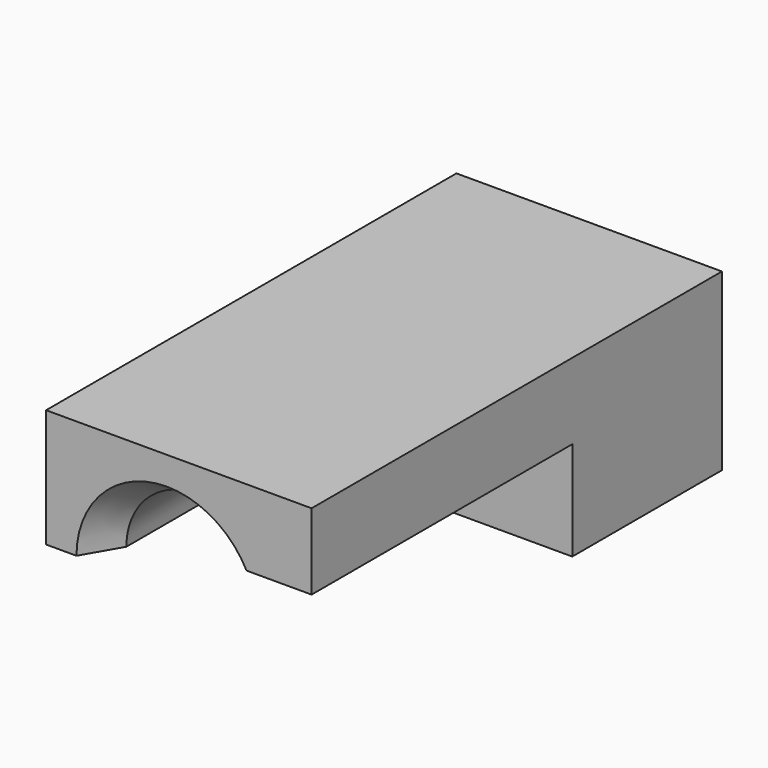
from build123d import *

# Parameters (mm, degrees)
F0_R     = 1.62
F0_R_2   = 2
F1_DEPTH = 15.5
F3_DEPTH = 27
F4_D     = 4
F4_DEPTH = 8
F4_TIP   = 1.2017212381
F5_DEPTH = 6
F6_SIZE2 = 1.7320508076
F6_SIZE  = 3


# Not quite as in the source:
# - ends of sketch curves that miss each other by under 0.0002 mm in the source are joined


with BuildPart() as f1:
    # F0 (on Front) → F1 (new body)
    with BuildSketch(Plane.XZ):
        with BuildLine():
            Line((-81.938941, 0.95), (-79.867763328, 0.95))
            ThreePointArc((-79.867763328, 0.95), (-84.599863166, 4.7050416476), (-90.5653650686, 3.7532564808))
            ThreePointArc((-90.5653650686, 3.7532564808), (-90.517166249, 3.503677095), (-90.501013, 3.25))
            ThreePointArc((-90.501013, 3.25), (-91.2509614327, 1.6887917887), (-92.9383840791, 1.2984092286))
            ThreePointArc((-92.9383840791, 1.2984092286), (-93.5417590804, 0.0341622689), (-93.899505073, -1.3202378094))
            ThreePointArc((-93.899505073, -1.3202378094), (-93.0082544766, -0.8153925244), (-91.9839548989, -0.8179930331))
            ThreePointArc((-91.9839548989, -0.8179930331), (-87.4977327048, 3.112954161), (-81.938941, 0.95))
        make_face()
        with BuildLine():
            ThreePointArc((-90.5653650686, 3.7532564808), (-84.599863166, 4.7050416476), (-79.867763328, 0.9499998269))
            Line((-79.867763328, 0.9499998269), (-74.501013, 0.95))
            Line((-74.501013, 0.95), (-74.501013, 7.25))
            Line((-74.501013, 7.25), (-96.501013, 7.25))
            Line((-96.501013, 7.25), (-96.501013, -2.55))
            Line((-96.501013, -2.55), (-94.4909878742, -2.55))
            ThreePointArc((-94.4909878742, -2.55), (-94.3033741804, -1.8831123628), (-93.899505073, -1.3202378094))
            ThreePointArc((-93.899505073, -1.3202378094), (-93.5417590804, 0.0341622689), (-92.9383840791, 1.2984092286))
            ThreePointArc((-92.9383840791, 1.2984092286), (-93.9389897521, 4.6400441937), (-90.5653650686, 3.7532564808))
        make_face()
        with Locations((-78.501013, 3.25)):
            Circle(F0_R, mode=Mode.SUBTRACT)
        with BuildLine():
            Line((-74.501013, 0.95), (-79.867763328, 0.95))
            Line((-79.867763328, 0.95), (-81.938941, 0.95))
            ThreePointArc((-81.9389410644, 0.9499999506), (-87.4977327048, 3.112954161), (-91.9839548989, -0.8179930331))
            ThreePointArc((-91.9839548989, -0.8179930331), (-92.0381964068, -1.0001290636), (-92.086389397, -1.1839580887))
            ThreePointArc((-92.086389397, -1.1839580887), (-91.2172509043, -1.7618932843), (-90.881013, -2.75))
            ThreePointArc((-90.881013, -2.75), (-92.6012048017, -4.3668987609), (-94.1086199171, -2.55))
            Line((-94.1086199171, -2.55), (-94.4909878742, -2.55))
            Line((-94.4909878742, -2.55), (-96.501013, -2.55))
            Line((-96.501013, -2.55), (-96.501013, -7.25))
            Line((-96.501013, -7.25), (-74.501013, -7.25))
            Line((-74.501013, -7.25), (-74.501013, 0.95))
        make_face()
        with Locations((-78.501013, -2.75)):
            Circle(F0_R_2, mode=Mode.SUBTRACT)
        with BuildLine():
            ThreePointArc((-92.9383840791, 1.2984092286), (-91.8934258204, 2.6626657264), (-90.5653650686, 3.7532564808))
            ThreePointArc((-90.5653650686, 3.7532564808), (-93.9389897521, 4.6400441937), (-92.9383840791, 1.2984092286))
        make_face()
        with Locations((-78.501013, -2.75)):
            Circle(F0_R_2)
        with BuildLine():
            ThreePointArc((-90.501013, 3.25), (-90.517166249, 3.503677095), (-90.5653650686, 3.7532564808))
            ThreePointArc((-90.5653650686, 3.7532564808), (-91.8934258204, 2.6626657264), (-92.9383840791, 1.2984092286))
            ThreePointArc((-92.9383840791, 1.2984092286), (-91.2509614327, 1.6887917887), (-90.501013, 3.25))
        make_face()
        with Locations((-78.501013, 3.25)):
            Circle(F0_R)
        with BuildLine():
            ThreePointArc((-93.9879149105, -2.1069426863), (-93.9540972375, -1.7124229299), (-93.899505073, -1.3202378094))
            ThreePointArc((-93.899505073, -1.3202378094), (-94.3033741804, -1.8831123628), (-94.4909878742, -2.55))
            Line((-94.4909878742, -2.55), (-94.1086199171, -2.55))
            ThreePointArc((-94.1086199171, -2.55), (-94.0640456826, -2.324172766), (-93.9879149105, -2.1069426863))
        make_face()
        with BuildLine():
            ThreePointArc((-92.086389397, -1.1839580887), (-92.0381964068, -1.0001290636), (-91.9839548989, -0.8179930331))
            ThreePointArc((-91.9839548989, -0.8179930331), (-93.0082544766, -0.8153925244), (-93.899505073, -1.3202378094))
            ThreePointArc((-93.899505073, -1.3202378094), (-93.9540972375, -1.7124229299), (-93.9879149105, -2.1069426863))
            ThreePointArc((-93.9879149105, -2.1069426863), (-93.2084169398, -1.29261204), (-92.086389397, -1.1839580887))
        make_face()
        with BuildLine():
            ThreePointArc((-90.881013, -2.75), (-91.2172509043, -1.7618932843), (-92.086389397, -1.1839580887))
            ThreePointArc((-92.086389397, -1.1839580887), (-92.2097087478, -1.8620371678), (-92.251013, -2.55))
            Line((-92.251013, -2.55), (-94.001013, -2.55))
            Line((-94.001013, -2.55), (-94.1086199171, -2.55))
            ThreePointArc((-94.1086199171, -2.55), (-92.6012048017, -4.3668987609), (-90.881013, -2.75))
        make_face()
        with BuildLine():
            ThreePointArc((-92.251013, -2.55), (-92.2097087478, -1.8620371678), (-92.086389397, -1.1839580887))
            ThreePointArc((-92.086389397, -1.1839580887), (-93.2084169398, -1.29261204), (-93.9879149105, -2.1069426863))
            ThreePointArc((-93.9879149105, -2.1069426863), (-93.9977377625, -2.3283745597), (-94.001013, -2.55))
            Line((-94.001013, -2.55), (-92.251013, -2.55))
        make_face()
        with BuildLine():
            ThreePointArc((-94.001013, -2.55), (-93.9977377625, -2.3283745597), (-93.9879149105, -2.1069426863))
            ThreePointArc((-93.9879149105, -2.1069426863), (-94.0640456826, -2.324172766), (-94.1086199171, -2.55))
            Line((-94.1086199171, -2.55), (-94.001013, -2.55))
        make_face()
    extrude(amount=F1_DEPTH)

    # F2 (on face) → F3 (join)
    with BuildSketch(Plane.XZ.offset(15.5)):
        with BuildLine():
            Line((-81.938941, 0.95), (-74.501013, 0.95))
            Line((-74.501013, 0.95), (-74.501013, 7.25))
            Line((-74.501013, 7.25), (-96.501013, 7.25))
            Line((-96.501013, 7.25), (-96.501013, -2.55))
            Line((-96.501013, -2.55), (-92.251013, -2.55))
            ThreePointArc((-92.251013, -2.55), (-88.3490641857, 2.8949248677), (-81.9389410644, 0.9499999506))
        make_face()
    extrude(amount=F3_DEPTH)

    # F4
    with Locations(Plane(origin=(0, 0, 0), x_dir=(1, 0, 0), z_dir=(0, 1, 0))):
        with Locations((-92.501013, 2.75), (-78.501013, -3.25)):
            Hole(F4_D / 2, depth=F4_DEPTH)
            with Locations((0, 0, -(F4_DEPTH + F4_TIP / 2))):  # 118° drill point
                Cone(0, F4_D / 2, F4_TIP, mode=Mode.SUBTRACT)

    # F0 (on Front) → F5 (cut)
    with BuildSketch(Plane.XZ):
        with BuildLine():
            ThreePointArc((-92.9383840791, 1.2984092286), (-91.8934258204, 2.6626657264), (-90.5653650686, 3.7532564808))
            ThreePointArc((-90.5653650686, 3.7532564808), (-93.9389897521, 4.6400441937), (-92.9383840791, 1.2984092286))
        make_face()
        with BuildLine():
            ThreePointArc((-90.501013, 3.25), (-90.517166249, 3.503677095), (-90.5653650686, 3.7532564808))
            ThreePointArc((-90.5653650686, 3.7532564808), (-91.8934258204, 2.6626657264), (-92.9383840791, 1.2984092286))
            ThreePointArc((-92.9383840791, 1.2984092286), (-91.2509614327, 1.6887917887), (-90.501013, 3.25))
        make_face()
        with Locations((-78.501013, -2.75)):
            Circle(F0_R_2)
    extrude(amount=F5_DEPTH, mode=Mode.SUBTRACT)

    # F6
    f6_edges = [f1.edges().sort_by_distance(p)[0] for p in [
        (-88.349064, -42.5, 2.894925),
    ]]
    f6_side = f1.faces().sort_by_distance((-88.349064, -29, 2.894925))[0]
    chamfer(f6_edges, length=F6_SIZE, length2=F6_SIZE2, reference=f6_side)


solid = f1.part
